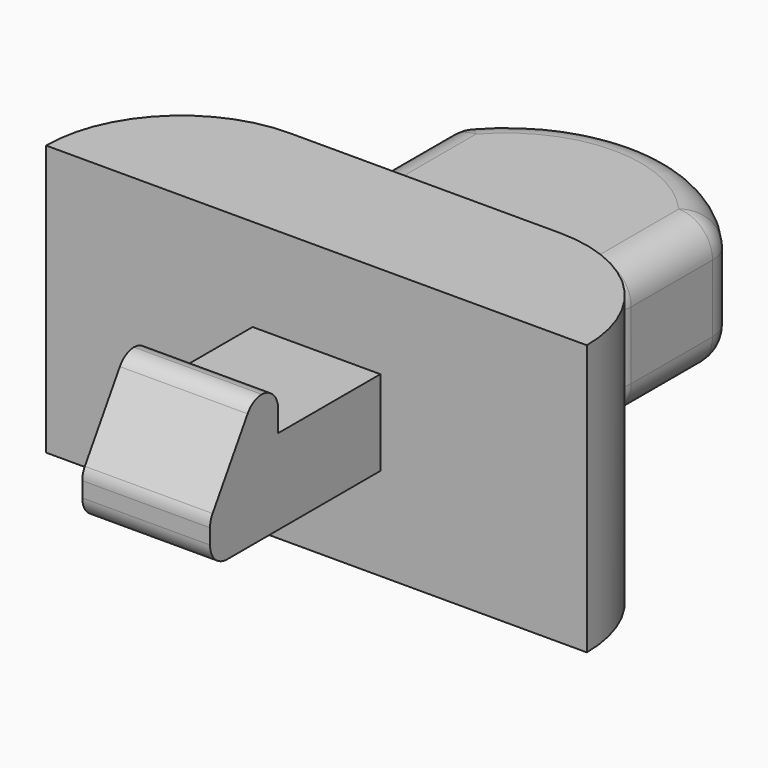
from build123d import *

# Parameters (mm, degrees)
F1_DEPTH    = 1.5875
F2_DEPTH    = 3.175
F3_R        = 3.17499
F4_R        = 0.79375
F5_R        = 0.508
F7_DEPTH    = 1.5
F8_T1_DEPTH = 5.5
F8_T3_DEPTH = 3.716990566
F8_T5_DEPTH = 4.3856191038


# Not quite as in the source:
# - a fillet or chamfer that OpenCascade refuses, or shapes differently, is made with other operations: its cross-section is extruded or revolved along the edge and cut away or added
# - a fillet or chamfer is up to 0.001 mm smaller than in the source, because OpenCascade refuses the exact size


with BuildPart() as f1:
    # F0 (on Top) → F1 (new body, symmetric)
    with BuildSketch(Plane.XY):
        with BuildLine():
            Line((3.175, 4.7625), (3.175, 7.9375))
            ThreePointArc((3.175, 7.9375), (0, 9.525), (-3.175, 7.9375))
            Line((-3.175, 7.9375), (-3.175, 4.7625))
            Line((-3.175, 4.7625), (-1.5875, 4.7625))
            Line((-1.5875, 4.7625), (-1.5875, 3.175))
            Line((-1.5875, 3.175), (1.5875, 3.175))
            Line((1.5875, 3.175), (1.5875, 4.7625))
            Line((1.5875, 4.7625), (3.175, 4.7625))
        make_face()
    extrude(amount=F1_DEPTH, both=True)

    # F0 (on Top) → F2 (join, symmetric)
    with BuildSketch(Plane.XY):
        Polygon((6.35, 3.175), (1.5875, 3.175), (-1.5875, 3.175), (-6.35, 3.175), (-6.35, 0), (6.35, 0), align=None)
    extrude(amount=F2_DEPTH, both=True)

    # F3 (radius 3.175 in the source; OpenCascade refuses exactly that, so slightly less here)
    f3_edges = [f1.edges().sort_by_distance(p)[0] for p in [
        (6.35, 3.175, 0),
        (-6.35, 3.175, 0),
    ]]
    fillet(f3_edges, radius=F3_R)

    # F4
    f4_edges = [f1.edges().sort_by_distance(p)[0] for p in [
        (0, 9.525, -1.5875),
        (0, 9.525, 1.5875),
        (3.175, 6.35, -1.5875),
        (3.175, 6.35, 1.5875),
        (-3.175, 6.35, -1.5875),
        (-3.175, 6.35, 1.5875),
        (3.175, 7.9375, 0),
        (-3.175, 7.9375, 0),
    ]]
    fillet(f4_edges, radius=F4_R)

    # F5
    f5_edges = [f1.edges().sort_by_distance(p)[0] for p in [
        (0, 3.175, -1.5875),
        (-1.5875, 3.175, 0),
        (0, 3.175, 1.5875),
        (1.5875, 3.175, 0),
        (1.5875, 3.96875, 1.5875),
        (1.5875, 3.96875, -1.5875),
        (-1.5875, 3.96875, -1.5875),
        (-1.5875, 3.96875, 1.5875),
        (2.942516, 4.7625, 1.355016),
        (-2.942516, 4.7625, -1.355016),
        (1.984375, 4.7625, -1.5875),
        (-1.984375, 4.7625, -1.5875),
        (2.942516, 4.7625, -1.355016),
        (3.175, 4.7625, 0),
        (1.984375, 4.7625, 1.5875),
        (-3.175, 4.7625, 0),
        (-2.942516, 4.7625, 1.355016),
        (-1.984375, 4.7625, 1.5875),
    ]]
    fillet(f5_edges, radius=F5_R)

    # F6 (on Right) → F7 (join, symmetric)
    with BuildSketch(Plane.YZ):
        Polygon((0, -1), (0, 1), (-3, 1), (-3, 2), (-3.75, 2), (-5, 0), (-5, -1), align=None)
    extrude(amount=F7_DEPTH, both=True)

    # F8: fillet of radius 0.5 on 4 edges, made by hand

    # F8_s2 → F8_t1 (cut)
    with BuildSketch(Plane.YZ.offset(-2.75)):
        with BuildLine():
            ThreePointArc((-4.5, -1), (-4.8535533906, -0.8535533906), (-5, -0.5))
            Line((-5, -0.5), (-5, -1))
            Line((-5, -1), (-4.5, -1))
        make_face()
        with BuildLine():
            ThreePointArc((-3, 1.5), (-3.1464466094, 1.8535533906), (-3.5, 2))
            Line((-3.5, 2), (-3, 2))
            Line((-3, 2), (-3, 1.5))
        make_face()
    extrude(amount=F8_T1_DEPTH, mode=Mode.SUBTRACT)

    # F8_s4 → F8_t3 (cut)
    with BuildSketch(Plane.YZ.offset(-1.858495283)):
        with BuildLine():
            ThreePointArc((-5, -0.1433981132), (-4.9806243731, -0.0055568567), (-4.923999152, 0.1216013568))
            Line((-4.923999152, 0.1216013568), (-5, 0))
            Line((-5, 0), (-5, -0.1433981132))
        make_face()
    extrude(amount=F8_T3_DEPTH, mode=Mode.SUBTRACT)

    # F8_s6 → F8_t5 (cut)
    with BuildSketch(Plane.YZ.offset(-2.1928095519)):
        with BuildLine():
            ThreePointArc((-3.4728761792, 2), (-3.7152604454, 1.9373212406), (-3.8968753312, 1.76499947))
            Line((-3.8968753312, 1.76499947), (-3.75, 2))
            Line((-3.75, 2), (-3.4728761792, 2))
        make_face()
    extrude(amount=F8_T5_DEPTH, mode=Mode.SUBTRACT)


solid = f1.part
